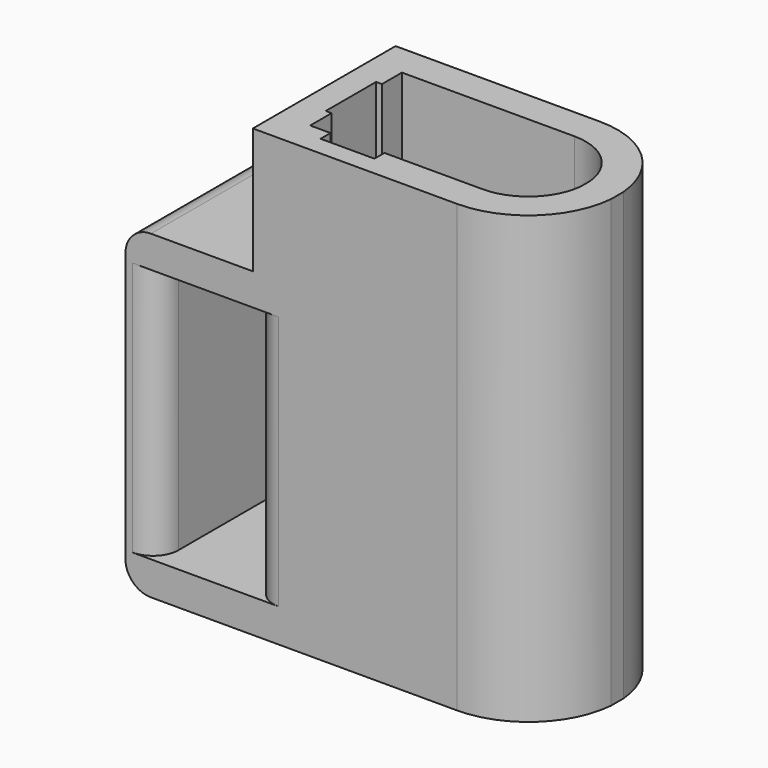
from build123d import *

# Parameters (mm, degrees)
F2_DEPTH  = 6.35
F3_DEPTH  = 25.4
F5_DEPTH  = 63.5
F6_W      = 35.5600007778
F6_H      = 6.6786579132
F7_DEPTH  = 25.4
F8_W      = 6.5081897405
F8_H      = 35.5600007778
F9_DEPTH  = 57.15
F10_W     = 35.5600007778
F10_H     = 6.35
F11_DEPTH = 19.05
F12_R     = 5.08
F13_R     = 5.08
F14_R     = 5.08
F15_R     = 5.08
F16_R     = 5.08


# Not quite as in the source:
# - two fillets or chamfers of one size are made in one step


with BuildPart() as f2:
    # F0 (on Top) → F2 (new body)
    with BuildSketch(Plane.XY):
        with BuildLine():
            ThreePointArc((-18.3481574059, -1.8204556262), (-18.2829820174, -0.6015784588), (-18.3481574059, 0.6172987085))
            Line((-18.3481574059, 0.6172987085), (-18.3481574059, -1.8204556262))
        make_face()
        with BuildLine():
            Line((-29.7129820174, 10.8284215412), (-64.0681574059, 10.8284215412))
            Line((-64.0681574059, 10.8284215412), (-64.0681574059, 5.8474093676))
            Line((-64.0681574059, 5.8474093676), (-65.235733552, 5.8474093676))
            Line((-65.235733552, 5.8474093676), (-65.235733552, -6.7013129592))
            Line((-65.235733552, -6.7013129592), (-64.0681574059, -6.7013129592))
            Line((-64.0681574059, -6.7013129592), (-64.0681574059, -12.0315784588))
            Line((-64.0681574059, -12.0315784588), (-60.0158534944, -12.0315784588))
            Line((-60.0158534944, -12.0315784588), (-60.0158534944, -14.5130921155))
            Line((-60.0158534944, -14.5130921155), (-49.2716534944, -14.5130921155))
            Line((-49.2716534944, -14.5130921155), (-49.2716534944, -12.0315784588))
            Line((-49.2716534944, -12.0315784588), (-29.7129820174, -12.0315784588))
            ThreePointArc((-29.7129820174, -12.0315784588), (-22.0738350108, -9.1038330429), (-18.3481574059, -1.8204556262))
            Line((-18.3481574059, -1.8204556262), (-18.3481574059, 0.6172987085))
            ThreePointArc((-18.3481574059, 0.6172987085), (-22.0738350108, 7.9006761252), (-29.7129820174, 10.8284215412))
        make_face()
    extrude(amount=-F2_DEPTH)

    # F1 (on Top) → F3 (join)
    with BuildSketch(Plane.XY):
        with BuildLine():
            Line((-42.9216531055, -18.3815788478), (-29.7129820174, -18.3815788478))
            ThreePointArc((-29.7129820174, -18.3815788478), (-17.6903920931, -13.7006526758), (-11.9981570169, -2.1225613757))
            Line((-11.9981570169, -2.1225613757), (-11.9981570169, 0.919404458))
            ThreePointArc((-11.9981570169, 0.919404458), (-17.6903920931, 12.4974957581), (-29.7129820174, 17.1784219301))
            Line((-29.7129820174, 17.1784219301), (-70.4181577948, 17.1784219301))
            Line((-70.4181577948, 17.1784219301), (-70.4181577948, 12.1974097565))
            Line((-70.4181577948, 12.1974097565), (-70.4181577948, -13.0513133481))
            Line((-70.4181577948, -13.0513133481), (-70.4181577948, -18.3815788478))
            Line((-70.4181577948, -18.3815788478), (-66.3658538833, -18.3815788478))
            Line((-66.3658538833, -18.3815788478), (-42.9216531055, -18.3815788478))
        make_face()
    extrude(amount=-F3_DEPTH)

    # F4 (on face) → F5 (join)
    with BuildSketch(Plane.XY):
        with BuildLine():
            Line((-42.9216538833, -18.3815788478), (-29.7129820174, -18.3815788478))
            ThreePointArc((-29.7129820174, -18.3815788478), (-17.6903920931, -13.7006526758), (-11.9981570169, -2.1225613757))
            Line((-11.9981570169, -2.1225613757), (-11.9981570169, 0.919404458))
            ThreePointArc((-11.9981570169, 0.919404458), (-17.6903920931, 12.4974957581), (-29.7129820174, 17.1784219301))
            Line((-29.7129820174, 17.1784219301), (-70.4181577948, 17.1784219301))
            Line((-70.4181577948, 17.1784219301), (-70.4181577948, 12.1974097565))
            Line((-70.4181577948, 12.1974097565), (-70.4181577948, -13.0513133481))
            Line((-70.4181577948, -13.0513133481), (-70.4181577948, -18.3815788478))
            Line((-70.4181577948, -18.3815788478), (-66.3658538833, -18.3815788478))
            Line((-66.3658538833, -18.3815788478), (-42.9216538833, -18.3815788478))
        make_face()
        with BuildLine():
            Line((-65.2357339409, 5.8474097565), (-64.0681577948, 5.8474097565))
            Line((-64.0681577948, 5.8474097565), (-64.0681577948, 10.8284219301))
            Line((-64.0681577948, 10.8284219301), (-29.7129820174, 10.8284219301))
            ThreePointArc((-29.7129820174, 10.8284219301), (-22.0738347431, 7.9006764075), (-18.3481570169, 0.6172987293))
            Line((-18.3481570169, 0.6172987293), (-18.3481570169, -1.820455647))
            ThreePointArc((-18.3481570169, -1.820455647), (-22.0738347431, -9.1038333252), (-29.7129820174, -12.0315788478))
            Line((-29.7129820174, -12.0315788478), (-49.2716531055, -12.0315788478))
            Line((-49.2716531055, -12.0315788478), (-49.2716531055, -14.5130925044))
            Line((-49.2716531055, -14.5130925044), (-60.0158538833, -14.5130925044))
            Line((-60.0158538833, -14.5130925044), (-60.0158538833, -12.0315788478))
            Line((-60.0158538833, -12.0315788478), (-64.0681577948, -12.0315788478))
            Line((-64.0681577948, -12.0315788478), (-64.0681577948, -6.7013133481))
            Line((-64.0681577948, -6.7013133481), (-65.2357339409, -6.7013133481))
            Line((-65.2357339409, -6.7013133481), (-65.2357339409, 5.8474097565))
        make_face(mode=Mode.SUBTRACT)
    extrude(amount=F5_DEPTH)

    # F6 (on face) → F7 (join)
    with BuildSketch(Plane(origin=(-70.4181577948, 0, 0), x_dir=(0, -1, 0), z_dir=(-1, 0, 0))):
        with Locations((0.6015784588, -22.0606710434)):
            Rectangle(F6_W, F6_H)
    extrude(amount=F7_DEPTH)

    # F8 (on face) → F9 (join)
    with BuildSketch(Plane.XY.offset(-18.7213420868)):
        with Locations((-92.5640629245, -0.6015784588)):
            Rectangle(F8_W, F8_H)
    extrude(amount=F9_DEPTH)

    # F10 (on face) → F11 (join)
    with BuildSketch(Plane.YZ.offset(-89.3099680543)):
        with Locations((-0.6015784588, 35.2536579132)):
            Rectangle(F10_W, F10_H)
    extrude(amount=F11_DEPTH)

    # F12
    f12_edges = [f2.edges().sort_by_distance(p)[0] for p in [
        (-95.818158, -0.601578, 38.428658),
    ]]
    fillet(f12_edges, radius=F12_R)

    # F13
    f13_edges = [f2.edges().sort_by_distance(p)[0] for p in [
        (-95.818158, -0.601578, -25.4),
    ]]
    fillet(f13_edges, radius=F13_R)

    # F14
    f14_edges = [f2.edges().sort_by_distance(p)[0] for p in [
        (-70.418158, -18.381579, 6.678658),
    ]]
    fillet(f14_edges, radius=F14_R)

    # F15
    f15_edges = [f2.edges().sort_by_distance(p)[0] for p in [
        (-70.418158, 17.178422, 6.678658),
    ]]
    fillet(f15_edges, radius=F15_R)

    # F16
    f16_edges = [f2.edges().sort_by_distance(p)[0] for p in [
        (-89.309968, 17.178422, 6.678658),
        (-89.309968, -18.381579, 6.678658),
    ]]
    fillet(f16_edges, radius=F16_R)


solid = f2.part
